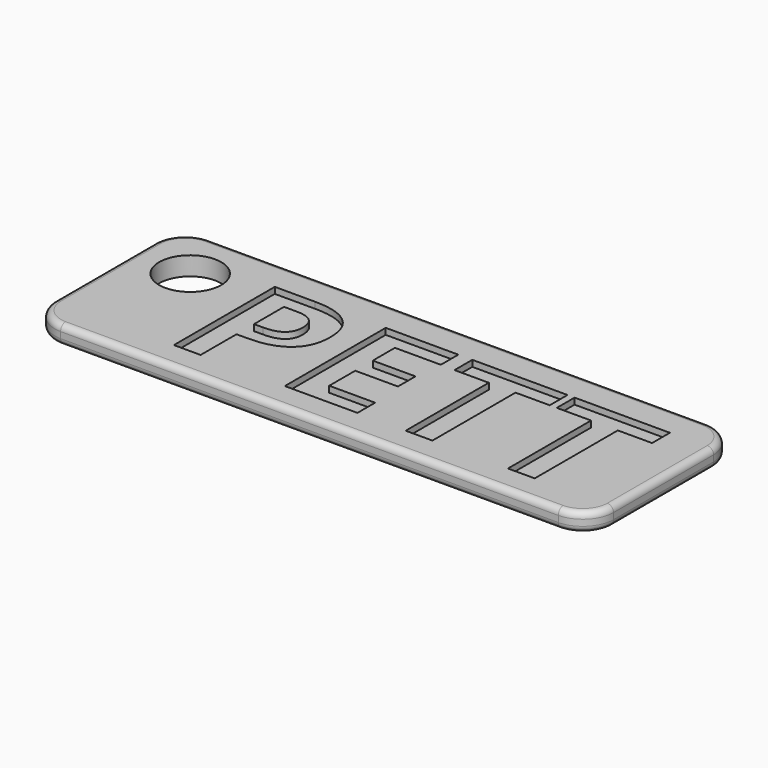
from build123d import *

# Parameters (mm, degrees)
F0_W         = 90
F0_H         = 30
F1_DEPTH     = 3
F2_R         = 1
F3_T1_DEPTH  = 3
F3_T4_ANGLE  = 90
F3_T6_ANGLE  = 90
F3_T8_ANGLE  = 90
F3_T10_ANGLE = 90
F3_T12_ANGLE = 90
F3_T14_ANGLE = 90
F3_T16_ANGLE = 90
F3_T18_ANGLE = 90
F4_R         = 5
F5_DEPTH     = 3
F6_TEXT_SIZE = 28.4407267024
F7_DEPTH     = 1


# Not quite as in the source:
# - a fillet or chamfer that OpenCascade refuses, or shapes differently, is made with other operations: its cross-section is extruded or revolved along the edge and cut away or added
# - Text() gives the source's letters only with a copy of the font that has no kerning and outlines rounded to 1/6400 em; it was checked with that copy


with BuildPart() as f1:
    # F0 (on Top) → F1 (new body)
    with BuildSketch(Plane.XY):
        Rectangle(F0_W, F0_H)
    extrude(amount=F1_DEPTH)

    # F2
    f2_edges = [f1.edges().sort_by_distance(p)[0] for p in [
        (0, 15, 3),
        (-45, 0, 3),
        (0, -15, 3),
        (45, 0, 3),
        (0, 15, 0),
        (-45, 0, 0),
        (0, -15, 0),
        (45, 0, 0),
    ]]
    fillet(f2_edges, radius=F2_R)

    # F3: fillet of radius 5 on 4 edges, made by hand

    # F3_s2 → F3_t1 (cut)
    with BuildSketch(Plane.XY):
        with BuildLine():
            ThreePointArc((45.0004, -9.9990343146), (43.5355339059, -13.5355339059), (39.9990343146, -15.0004))
            Line((39.9990343146, -15.0004), (39.9990343146, -15.5005365685))
            ThreePointArc((39.9990343146, -15.5005365685), (42.4995171573, -15.5001365685), (45, -15.5001365685))
            Line((45, -15.5001365685), (45.5001365685, -15))
            ThreePointArc((45.5001365685, -15), (45.5001365685, -12.4995171573), (45.5005365685, -9.9990343146))
            Line((45.5005365685, -9.9990343146), (45.0004, -9.9990343146))
        make_face()
        with BuildLine():
            ThreePointArc((39.9990343146, 15.0004), (43.5355339059, 13.5355339059), (45.0004, 9.9990343146))
            Line((45.0004, 9.9990343146), (45.5005365685, 9.9990343146))
            ThreePointArc((45.5005365685, 9.9990343146), (45.5001365685, 12.4995171573), (45.5001365685, 15))
            Line((45.5001365685, 15), (45, 15.5001365685))
            ThreePointArc((45, 15.5001365685), (42.4995171573, 15.5001365685), (39.9990343146, 15.5005365685))
            Line((39.9990343146, 15.5005365685), (39.9990343146, 15.0004))
        make_face()
        with BuildLine():
            ThreePointArc((-39.9990343146, 15.0004), (-43.5355339059, 13.5355339059), (-45.0004, 9.9990343146))
            Line((-45.0004, 9.9990343146), (-45.5005365685, 9.9990343146))
            ThreePointArc((-45.5005365685, 9.9990343146), (-45.5001365685, 12.4995171573), (-45.5001365685, 15))
            Line((-45.5001365685, 15), (-45, 15.5001365685))
            ThreePointArc((-45, 15.5001365685), (-42.4995171573, 15.5001365685), (-39.9990343146, 15.5005365685))
            Line((-39.9990343146, 15.5005365685), (-39.9990343146, 15.0004))
        make_face()
        with BuildLine():
            ThreePointArc((-45.0004, -9.9990343146), (-43.5355339059, -13.5355339059), (-39.9990343146, -15.0004))
            Line((-39.9990343146, -15.0004), (-39.9990343146, -15.5005365685))
            ThreePointArc((-39.9990343146, -15.5005365685), (-42.4995171573, -15.5001365685), (-45, -15.5001365685))
            Line((-45, -15.5001365685), (-45.5001365685, -15))
            ThreePointArc((-45.5001365685, -15), (-45.5001365685, -12.4995171573), (-45.5005365685, -9.9990343146))
            Line((-45.5005365685, -9.9990343146), (-45.0004, -9.9990343146))
        make_face()
    extrude(amount=F3_T1_DEPTH, mode=Mode.SUBTRACT)

    # F3_s3 → F3_t4 (revolve, cut)
    with BuildSketch(Plane.YZ.offset(-39.9990343146)):
        with BuildLine():
            ThreePointArc((-14.0004, 0), (-14.7075067812, 0.2928932188), (-15.0004, 1))
            Line((-15.0004, 1), (-15.0004, 0))
            Line((-15.0004, 0), (-14.0004, 0))
        make_face()
    revolve(axis=Axis((-39.9990343146, -9.9990343146, 0), (0, 0, -1)), revolution_arc=F3_T4_ANGLE, mode=Mode.SUBTRACT)

    # F3_s5 → F3_t6 (revolve, cut)
    with BuildSketch(Plane.XZ.offset(9.9990343146)):
        with BuildLine():
            ThreePointArc((-44.0004, 3), (-44.7075067812, 2.7071067812), (-45.0004, 2))
            Line((-45.0004, 2), (-45.0004, 3))
            Line((-45.0004, 3), (-44.0004, 3))
        make_face()
    revolve(axis=Axis((-39.9990343146, -9.9990343146, 3), (0, 0, 1)), revolution_arc=F3_T6_ANGLE, mode=Mode.SUBTRACT)

    # F3_s7 → F3_t8 (revolve, cut)
    with BuildSketch(Plane.XZ.offset(-9.9990343146)):
        with BuildLine():
            ThreePointArc((-44.0004, 0), (-44.7075067812, 0.2928932188), (-45.0004, 1))
            Line((-45.0004, 1), (-45.0004, 0))
            Line((-45.0004, 0), (-44.0004, 0))
        make_face()
    revolve(axis=Axis((-39.9990343146, 9.9990343146, 0), (0, 0, -1)), revolution_arc=F3_T8_ANGLE, mode=Mode.SUBTRACT)

    # F3_s9 → F3_t10 (revolve, cut)
    with BuildSketch(Plane.YZ.offset(-39.9990343146)):
        with BuildLine():
            ThreePointArc((14.0004, 3), (14.7075067812, 2.7071067812), (15.0004, 2))
            Line((15.0004, 2), (15.0004, 3))
            Line((15.0004, 3), (14.0004, 3))
        make_face()
    revolve(axis=Axis((-39.9990343146, 9.9990343146, 3), (0, 0, 1)), revolution_arc=F3_T10_ANGLE, mode=Mode.SUBTRACT)

    # F3_s11 → F3_t12 (revolve, cut)
    with BuildSketch(Plane.YZ.offset(39.9990343146)):
        with BuildLine():
            ThreePointArc((14.0004, 0), (14.7075067812, 0.2928932188), (15.0004, 1))
            Line((15.0004, 1), (15.0004, 0))
            Line((15.0004, 0), (14.0004, 0))
        make_face()
    revolve(axis=Axis((39.9990343146, 9.9990343146, 0), (0, 0, -1)), revolution_arc=F3_T12_ANGLE, mode=Mode.SUBTRACT)

    # F3_s13 → F3_t14 (revolve, cut)
    with BuildSketch(Plane.XZ.offset(-9.9990343146)):
        with BuildLine():
            ThreePointArc((44.0004, 3), (44.7075067812, 2.7071067812), (45.0004, 2))
            Line((45.0004, 2), (45.0004, 3))
            Line((45.0004, 3), (44.0004, 3))
        make_face()
    revolve(axis=Axis((39.9990343146, 9.9990343146, 3), (0, 0, 1)), revolution_arc=F3_T14_ANGLE, mode=Mode.SUBTRACT)

    # F3_s15 → F3_t16 (revolve, cut)
    with BuildSketch(Plane.XZ.offset(9.9990343146)):
        with BuildLine():
            ThreePointArc((44.0004, 0), (44.7075067812, 0.2928932188), (45.0004, 1))
            Line((45.0004, 1), (45.0004, 0))
            Line((45.0004, 0), (44.0004, 0))
        make_face()
    revolve(axis=Axis((39.9990343146, -9.9990343146, 0), (0, 0, -1)), revolution_arc=F3_T16_ANGLE, mode=Mode.SUBTRACT)

    # F3_s17 → F3_t18 (revolve, cut)
    with BuildSketch(Plane.YZ.offset(39.9990343146)):
        with BuildLine():
            ThreePointArc((-14.0004, 3), (-14.7075067812, 2.7071067812), (-15.0004, 2))
            Line((-15.0004, 2), (-15.0004, 3))
            Line((-15.0004, 3), (-14.0004, 3))
        make_face()
    revolve(axis=Axis((39.9990343146, -9.9990343146, 3), (0, 0, 1)), revolution_arc=F3_T18_ANGLE, mode=Mode.SUBTRACT)

    # F4 (on face) → F5 (cut)
    with BuildSketch(Plane.XY.offset(3)):
        with Locations((-36, 6)):
            Circle(F4_R)
    extrude(amount=-F5_DEPTH, mode=Mode.SUBTRACT)

    # F6 (on face) → F7 (cut)
    with BuildSketch(Plane.XY.offset(3)):
        with Locations((-28, -10.4773232257)):
            Text('PETT', F6_TEXT_SIZE, font='Open Sans', font_style=FontStyle.BOLD, text_align=(TextAlign.LEFT, TextAlign.BOTTOM))
    extrude(amount=-F7_DEPTH, mode=Mode.SUBTRACT)


solid = f1.part
